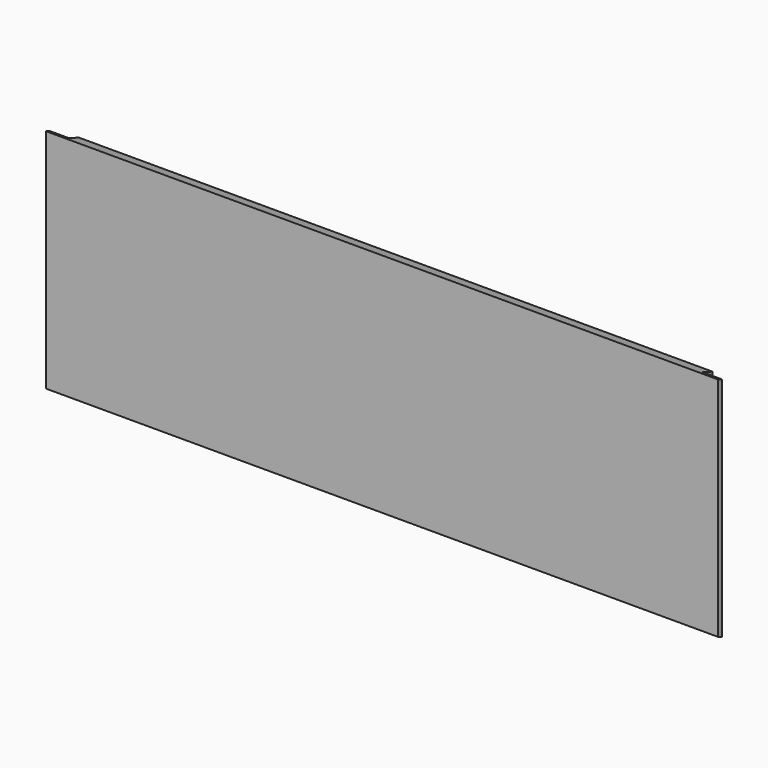
from build123d import *

# Parameters (mm, degrees)
F0_W       = 875
F0_H       = 303
F1_DEPTH   = 22
F2_SIZE2   = 8.007335
F2_SIZE    = 21.99999
F2_2_SIZE2 = 8.007335
F2_2_SIZE  = 21.99999
F3_W       = 25
F3_H       = 16
F4_DEPTH   = 200


# Not quite as in the source:
# - a fillet or chamfer is up to 0.001 mm smaller than in the source, because OpenCascade refuses the exact size


with BuildPart() as f1:
    # F0 (on Front) → F1 (new body)
    with BuildSketch(Plane.XZ):
        Rectangle(F0_W, F0_H)
    extrude(amount=F1_DEPTH)

    # F2 (size 22 and 8.0073451539 in the source; OpenCascade refuses exactly that, so slightly less here)
    f2_edges = [f1.edges().sort_by_distance(p)[0] for p in [
        (0, -22, -151.5),
    ]]
    f2_side = f1.faces().sort_by_distance((0, -11, -151.5))[0]
    chamfer(f2_edges, length=F2_SIZE, length2=F2_SIZE2, reference=f2_side)

    # F2#2 (size 22 and 8.0073451539 in the source; OpenCascade refuses exactly that, so slightly less here)
    f2_2_edges = [f1.edges().sort_by_distance(p)[0] for p in [
        (0, 0, 151.5),
    ]]
    f2_2_side = f1.faces().sort_by_distance((0, -11, 151.5))[0]
    chamfer(f2_2_edges, length=F2_2_SIZE, length2=F2_2_SIZE2, reference=f2_2_side)

    # F3 (on Top) → F4 (cut, symmetric)
    with BuildSketch(Plane.XY):
        with Locations((425, -8)):
            Rectangle(F3_W, F3_H)
        with Locations((-425, -8)):
            Rectangle(F3_W, F3_H)
    extrude(amount=F4_DEPTH, both=True, mode=Mode.SUBTRACT)


solid = f1.part
